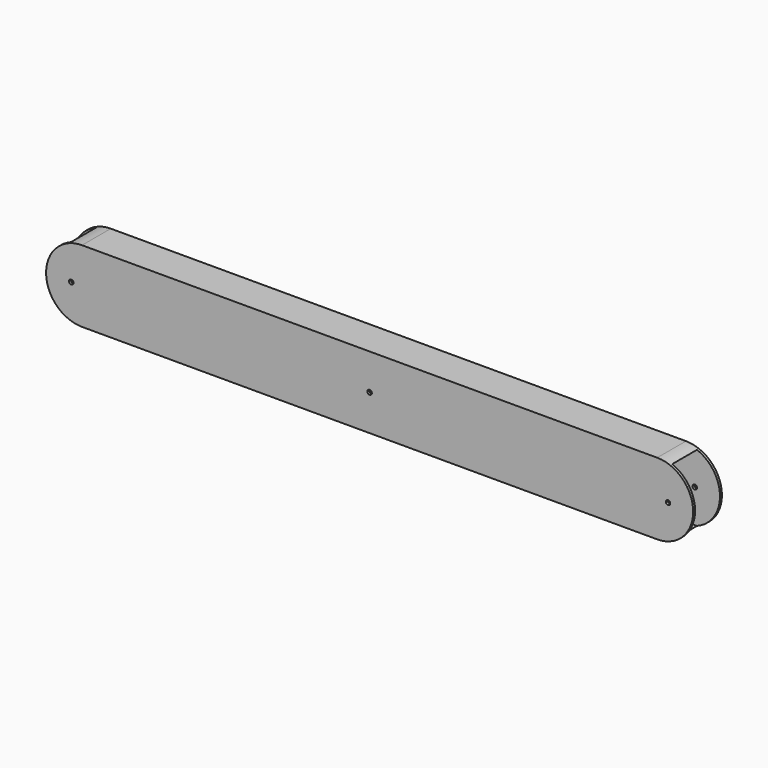
from build123d import *

# Parameters (mm, degrees)
F0_W        = 25.4
F0_H        = 50.8
F1_DEPTH    = 228.6
F2_W        = 21.971
F2_H        = 47.371
F3_DEPTH    = 457.201
F4_R        = 1.5875
F5_DEPTH    = 25.401
F6_R        = 1.5875
F7_DEPTH    = 25.401
F8_T1_DEPTH = 152.4
F9_T1_DEPTH = 152.4


# Not quite as in the source:
# - a fillet or chamfer that OpenCascade refuses, or shapes differently, is made with other operations: its cross-section is extruded or revolved along the edge and cut away or added


with BuildPart() as f1:
    # F0 (on Right) → F1 (new body, symmetric)
    with BuildSketch(Plane.YZ):
        Rectangle(F0_W, F0_H)
    extrude(amount=F1_DEPTH, both=True)

    # F2 (on face) → F3 (cut, through all)
    with BuildSketch(Plane.YZ.offset(228.6)):
        Rectangle(F2_W, F2_H)
    extrude(amount=-F3_DEPTH, mode=Mode.SUBTRACT)

    # F4 (on face) → F5 (cut, through all)
    with BuildSketch(Plane.XZ.offset(12.7)):
        with Locations((-210.82, 0)):
            Circle(F4_R)
        Circle(F4_R)
    extrude(amount=-F5_DEPTH, mode=Mode.SUBTRACT)

    # F6 (on face) → F7 (cut, through all)
    with BuildSketch(Plane.XZ.offset(12.7)):
        with Locations((210.82, 0)):
            Circle(F6_R)
    extrude(amount=-F7_DEPTH, mode=Mode.SUBTRACT)

    # F8: fillet of radius 25.4 on 2 edges, made by hand

    # F8_s2 → F8_t1 (cut)
    with BuildSketch(Plane.XZ.offset(-76.2)):
        with BuildLine():
            ThreePointArc((-228.6, 0), (-221.1605122421, -17.9605122421), (-203.2, -25.4))
            Line((-203.2, -25.4), (-228.6, -25.4))
            Line((-228.6, -25.4), (-228.6, 0))
        make_face()
        with BuildLine():
            ThreePointArc((-228.6, 0), (-221.1605122421, 17.9605122421), (-203.2, 25.4))
            Line((-203.2, 25.4), (-228.6, 25.4))
            Line((-228.6, 25.4), (-228.6, 0))
        make_face()
    extrude(amount=F8_T1_DEPTH, mode=Mode.SUBTRACT)

    # F9: fillet of radius 25.4 on 2 edges, made by hand

    # F9_s2 → F9_t1 (cut)
    with BuildSketch(Plane.XZ.offset(-76.2)):
        with BuildLine():
            ThreePointArc((203.2, 25.4), (221.1605122421, 17.9605122421), (228.6, 0))
            Line((228.6, 0), (228.6, 25.4))
            Line((228.6, 25.4), (203.2, 25.4))
        make_face()
        with BuildLine():
            ThreePointArc((228.6, 0), (221.1605122421, -17.9605122421), (203.2, -25.4))
            Line((203.2, -25.4), (228.6, -25.4))
            Line((228.6, -25.4), (228.6, 0))
        make_face()
    extrude(amount=F9_T1_DEPTH, mode=Mode.SUBTRACT)


solid = f1.part
